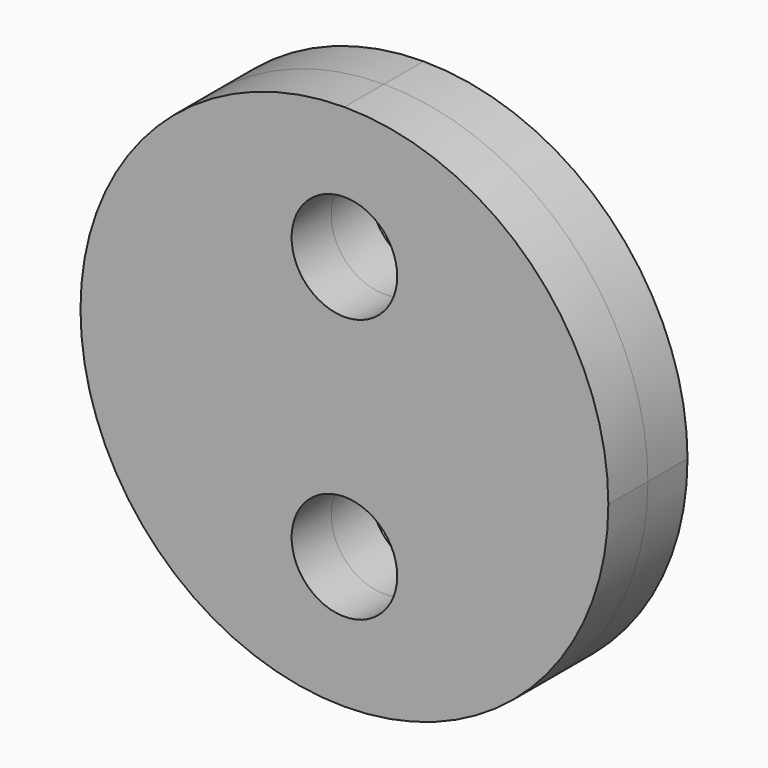
from build123d import *

# Parameters (mm, degrees)
F0_R     = 8
F1_DEPTH = 7.5


# Not quite as in the source:
# - the program builds the solid bodies; features that only make, move or delete a surface that nothing else refers to are left out


with BuildPart() as f1:
    # F0 (on Front) → F1 (new body, symmetric)
    with BuildSketch(Plane.XZ):
        with BuildLine():
            ThreePointArc((0, -40), (28.2842712475, -28.2842712475), (40, 0))
            ThreePointArc((40, 0), (28.2842712475, 28.2842712475), (0, 40))
            ThreePointArc((0, 40), (-20, 20), (0, 0))
            ThreePointArc((0, 0), (20, -20), (0, -40))
        make_face()
        with Locations((0, 20)):
            Circle(F0_R, mode=Mode.SUBTRACT)
        with BuildLine():
            ThreePointArc((0, 0), (-20, 20), (0, 40))
            ThreePointArc((0, 40), (-40, 0), (0, -40))
            ThreePointArc((0, -40), (20, -20), (0, 0))
        make_face()
        with Locations((0, -20)):
            Circle(F0_R, mode=Mode.SUBTRACT)
    extrude(amount=F1_DEPTH, both=True)


solid = f1.part
